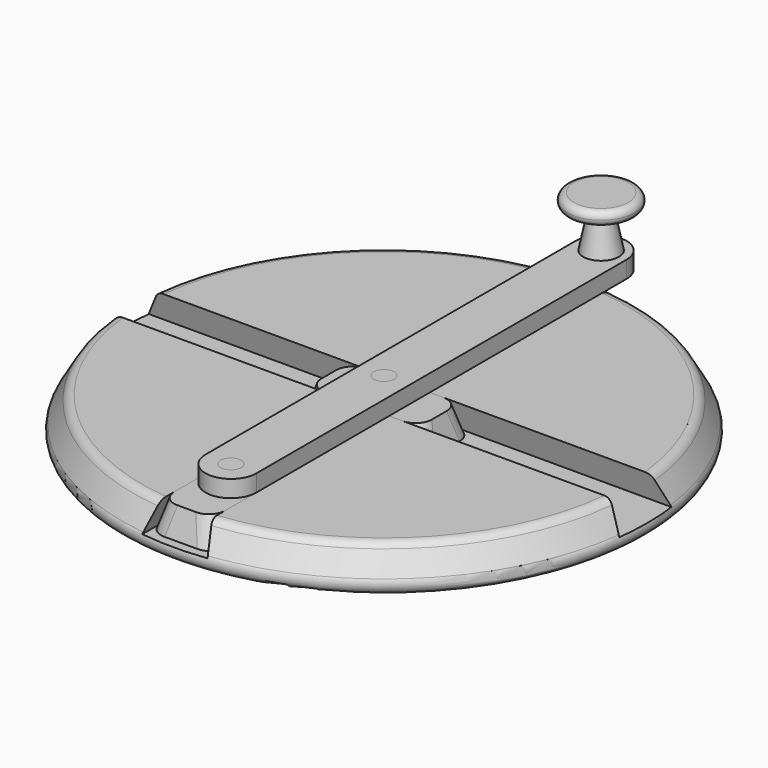
from build123d import *

# Parameters (mm, degrees)
F0_R          = 80
F1_DEPTH      = 12
F1_TAPER      = 30
F2_W          = 15
F2_H          = 72.1476616104
F2_H_2        = 15
F2_W_2        = 72.1476616104
F3_DEPTH      = 8
F3_TAPER      = -15
F4_W          = 15
F4_H          = 32.5929411411
F5_DEPTH      = 8
F5_TAPER      = -15
F4_W_2        = 32.5929411411
F4_H_2        = 15
F6_R          = 3
F7_DEPTH      = 5
F8_R          = 3
F9_DEPTH      = 5
F13_R         = 5
F13_2_R       = 5
F14_T4_ANGLE  = 85.0103001917
F14_T6_ANGLE  = 85.0103001917
F14_T8_ANGLE  = 85.0103001917
F14_T10_ANGLE = 85.0103001917


# Not quite as in the source:
# - a fillet or chamfer that OpenCascade refuses, or shapes differently, is made with other operations: its cross-section is extruded or revolved along the edge and cut away or added


with BuildPart() as f1:
    # F0 (on Top) → F1 (new body)
    with BuildSketch(Plane.XY):
        Circle(F0_R)
    extrude(amount=F1_DEPTH, taper=F1_TAPER)

    # F2 (on face) → F3 (cut)
    with BuildSketch(Plane.XY.offset(12)):
        with Locations((0, -43.5738308052)):
            Rectangle(F2_W, F2_H)
        Rectangle(F2_W, F2_H_2)
        with Locations((43.5738308052, 0)):
            Rectangle(F2_W_2, F2_H_2)
        with Locations((-43.5738308052, 0)):
            Rectangle(F2_W_2, F2_H_2)
        with Locations((0, 43.5738308052)):
            Rectangle(F2_W, F2_H)
    extrude(amount=-F3_DEPTH, taper=F3_TAPER, mode=Mode.SUBTRACT)

    # F14: fillet of radius 3 on 5 edges, made by hand

    # F14_s1 → F14_t2 (revolve, cut)
    with BuildSketch(Plane.XZ):
        with BuildLine():
            ThreePointArc((74.8038475773, 0), (77.4019237886, 1.5), (77.4019237886, 4.5))
            Line((77.4019237886, 4.5), (80, 0))
            Line((80, 0), (74.8038475773, 0))
        make_face()
    revolve(axis=Axis((0, 0, 0), (0, 0, -1)), mode=Mode.SUBTRACT)

    # F14_s3 → F14_t4 (revolve, cut)
    with BuildSketch(Plane(origin=(0, 0, 0), x_dir=(0, 0, 1), z_dir=(0.9990521383, -0.0435295866, 0))):
        with BuildLine():
            ThreePointArc((10.5, 73.9378221735), (11.5980762114, 72.8397459622), (12, 71.3397459622))
            Line((12, 71.3397459622), (12, 73.0717967697))
            Line((12, 73.0717967697), (10.5, 73.9378221735))
        make_face()
    revolve(axis=Axis((0, 0, 12), (0, 0, -1)), revolution_arc=F14_T4_ANGLE, mode=Mode.SUBTRACT)

    # F14_s5 → F14_t6 (revolve, cut)
    with BuildSketch(Plane(origin=(0, 0, 0), x_dir=(0, 0, 1), z_dir=(-0.0435295866, -0.9990521383, 0))):
        with BuildLine():
            ThreePointArc((10.5, 73.9378221735), (11.5980762114, 72.8397459622), (12, 71.3397459622))
            Line((12, 71.3397459622), (12, 73.0717967697))
            Line((12, 73.0717967697), (10.5, 73.9378221735))
        make_face()
    revolve(axis=Axis((0, 0, 12), (0, 0, -1)), revolution_arc=F14_T6_ANGLE, mode=Mode.SUBTRACT)

    # F14_s7 → F14_t8 (revolve, cut)
    with BuildSketch(Plane(origin=(0, 0, 0), x_dir=(0, 0, 1), z_dir=(-0.9990521383, 0.0435295866, 0))):
        with BuildLine():
            ThreePointArc((10.5, 73.9378221735), (11.5980762114, 72.8397459622), (12, 71.3397459622))
            Line((12, 71.3397459622), (12, 73.0717967697))
            Line((12, 73.0717967697), (10.5, 73.9378221735))
        make_face()
    revolve(axis=Axis((0, 0, 12), (0, 0, -1)), revolution_arc=F14_T8_ANGLE, mode=Mode.SUBTRACT)

    # F14_s9 → F14_t10 (revolve, cut)
    with BuildSketch(Plane(origin=(0, 0, 0), x_dir=(0, 0, 1), z_dir=(0.0435295866, 0.9990521383, 0))):
        with BuildLine():
            ThreePointArc((10.5, 73.9378221735), (11.5980762114, 72.8397459622), (12, 71.3397459622))
            Line((12, 71.3397459622), (12, 73.0717967697))
            Line((12, 73.0717967697), (10.5, 73.9378221735))
        make_face()
    revolve(axis=Axis((0, 0, 12), (0, 0, -1)), revolution_arc=F14_T10_ANGLE, mode=Mode.SUBTRACT)


with BuildPart() as f5:
    # F4 (on face) → F5 (new body)
    with BuildSketch(Plane.XY.offset(12)):
        with Locations((0, -56.3894117117)):
            Rectangle(F4_W, F4_H)
    extrude(amount=-F5_DEPTH, taper=F5_TAPER)

    # F6 (on face) → F7, piece 2 (join)
    with BuildSketch(Plane.XY.offset(12)):
        with Locations((0, -56.3894117117)):
            Circle(F6_R)
    extrude(amount=F7_DEPTH)

    # F13
    f13_edges = [f5.edges().sort_by_distance(p)[0] for p in [
        (-8.571797, -73.757679, 8),
        (8.571797, -73.757679, 8),
        (8.571797, -39.021144, 8),
        (-8.571797, -39.021144, 8),
    ]]
    fillet(f13_edges, radius=F13_R)


with BuildPart() as f5b:
    # F4 (on face) → F5, piece 2 (new body)
    with BuildSketch(Plane.XY.offset(12)):
        Rectangle(F4_W_2, F4_H_2)
    extrude(amount=-F5_DEPTH, taper=F5_TAPER)

    # F6 (on face) → F7 (join)
    with BuildSketch(Plane.XY.offset(12)):
        Circle(F6_R)
    extrude(amount=F7_DEPTH)

    # F13#2
    f13_2_edges = [f5b.edges().sort_by_distance(p)[0] for p in [
        (-17.368267, -8.571797, 8),
        (17.368267, -8.571797, 8),
        (17.368267, 8.571797, 8),
        (-17.368267, 8.571797, 8),
    ]]
    fillet(f13_2_edges, radius=F13_2_R)


with BuildPart() as f9:
    # F8 (on face) → F9 (new body, through all)
    with BuildSketch(Plane.XY.offset(12)):
        with BuildLine():
            ThreePointArc((-7.5, -56.3894117117), (0, -63.8894117117), (7.5, -56.3894117117))
            Line((7.5, -56.3894117117), (7.5, 80))
            ThreePointArc((7.5, 80), (0, 87.5), (-7.5, 80))
            Line((-7.5, 80), (-7.5, -56.3894117117))
        make_face()
        with Locations((0, -56.3894117117)):
            Circle(F8_R, mode=Mode.SUBTRACT)
        Circle(F8_R, mode=Mode.SUBTRACT)
        with Locations((0, 80)):
            Circle(F8_R, mode=Mode.SUBTRACT)
    extrude(amount=F9_DEPTH)


with BuildPart() as f12:
    # F11 (on plane+point) → F12 (revolve)
    with BuildSketch(Plane.XZ.offset(-80)):
        with BuildLine():
            Line((-3, 17), (-3, 12))
            Line((-3, 12), (0, 12))
            Line((0, 12), (0, 32))
            Line((0, 32), (-8, 32))
            ThreePointArc((-8, 32), (-9.4142135623, 31.4142135623), (-10, 30))
            ThreePointArc((-10, 30), (-9.4142135624, 28.5857864376), (-8, 28))
            Line((-8, 28), (-5.4505010521, 28))
            ThreePointArc((-5.4505010521, 28), (-3.9010519654, 27.2645977731), (-3.4910711875, 25.5992075277))
            Line((-3.4910711875, 25.5992075277), (-5.25, 17))
            Line((-5.25, 17), (-3, 17))
        make_face()
    revolve(axis=Axis((0, 80, 22), (0, 0, 1)))


solid = Compound([f1.part, f5.part, f5b.part, f9.part, f12.part])
